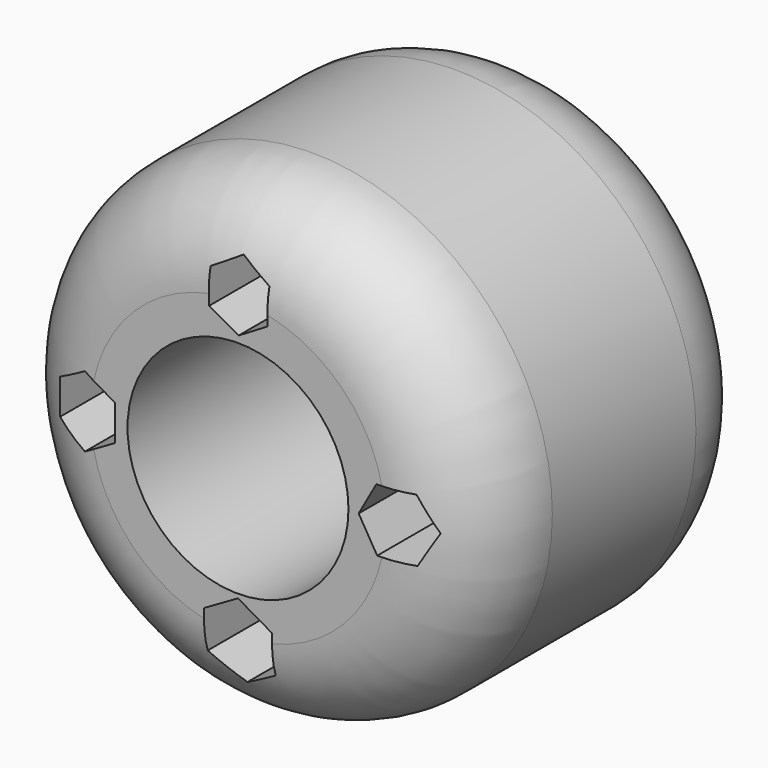
from build123d import *

# Parameters (mm, degrees)
F0_R     = 5
F0_R_2   = 2.3
F1_DEPTH = 3.8


# Not quite as in the source:
# - a fillet or chamfer that OpenCascade refuses, or shapes differently, is made with other operations: its cross-section is extruded or revolved along the edge and cut away or added


with BuildPart() as f1:
    # F0 (on Front) → F1 (new body, symmetric)
    with BuildSketch(Plane.XZ):
        Circle(F0_R)
        Polygon((0, -4.0174636819), (-0.7082950324, -3.6085293543), (-0.7082950324, -2.7906606991), (0, -2.3817263714), (0.7082950324, -2.7906606991), (0.7082950324, -3.6085293543), align=None, mode=Mode.SUBTRACT)
        Polygon((-3.1964122335, 0.7368465077), (-2.5582844391, 0.3684232539), (-2.5582844391, -0.3684232539), (-3.1964122335, -0.7368465077), (-3.8345400279, -0.3684232539), (-3.8345400279, 0.3684232539), align=None, mode=Mode.SUBTRACT)
        Circle(F0_R_2, mode=Mode.SUBTRACT)
        Polygon((2.8982667587, -0.6579181574), (2.512562897, -0.0101405277), (2.8807028495, 0.6477776297), (3.6345466637, 0.6579181574), (4.0202505254, 0.0101405277), (3.6521105729, -0.6477776297), align=None, mode=Mode.SUBTRACT)
        Polygon((0.6046901305, 3.5066245139), (0.6168706685, 2.8013560578), (0.012180538, 2.4381731744), (-0.6046901305, 2.7802587472), (-0.6168706685, 3.4855272032), (-0.012180538, 3.8487100866), align=None, mode=Mode.SUBTRACT)
    extrude(amount=F1_DEPTH, both=True)

    # F2: fillet of radius 1.9313708499 on 3 edges, made by hand

    # F2_s1 → F2_t2 (revolve, cut)
    with BuildSketch(Plane.XY):
        with BuildLine():
            ThreePointArc((5, 1.8686291501), (4.4343145751, 3.2343145751), (3.0686291501, 3.8))
            Line((3.0686291501, 3.8), (5, 3.8))
            Line((5, 3.8), (5, 1.8686291501))
        make_face()
    revolve(axis=Axis((0, 3.8, 0), (0, -1, 0)), mode=Mode.SUBTRACT)

    # F2_s3 → F2_t4 (revolve, cut)
    with BuildSketch(Plane.XY):
        with BuildLine():
            ThreePointArc((5, -1.8686291501), (4.4343145751, -3.2343145751), (3.0686291501, -3.8))
            Line((3.0686291501, -3.8), (5, -3.8))
            Line((5, -3.8), (5, -1.8686291501))
        make_face()
    revolve(axis=Axis((0, -3.8, 0), (0, -1, 0)), mode=Mode.SUBTRACT)


solid = f1.part
